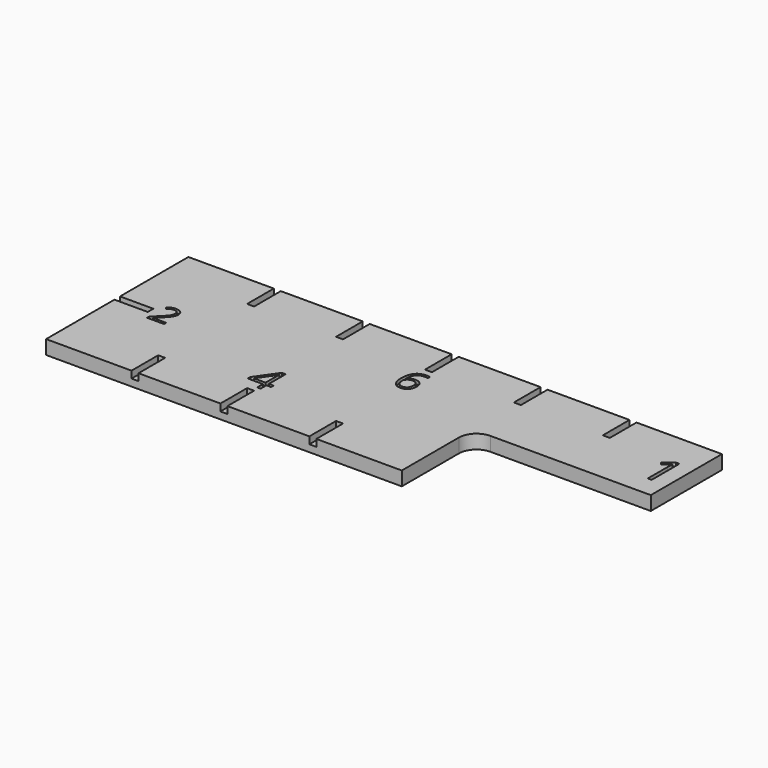
from build123d import *

# Parameters (mm, degrees)
F1_DEPTH       = 4
F3_DEPTH       = 2
F4_TEXT_SIZE   = 10.261640677
F4_TEXT_SIZE_2 = 11.3518313608
F4_TEXT_SIZE_3 = 12.4870120392
F4_TEXT_SIZE_4 = 13.8751825576
F5_DEPTH       = 1


# Not quite as in the source:
# - Text() gives the source's letters only with a copy of the font that has no kerning and outlines rounded to 1/6400 em; it was checked with that copy


with BuildPart() as f1:
    # F0 (on Top) → F1 (new body)
    with BuildSketch(Plane.XY):
        with BuildLine():
            Line((50.8, 25.4), (-50.8, 25.4))
            Line((-50.8, 25.4), (-50.8, -25.4))
            Line((-50.8, -25.4), (50.8, -25.4))
            Line((50.8, -25.4), (50.8, -5))
            ThreePointArc((50.8, -5), (52.2644660941, -1.4644660941), (55.8, 0))
            Line((55.8, 0), (101.6, 0))
            Line((101.6, 0), (101.6, 25.4))
            Line((101.6, 25.4), (50.8, 25.4))
        make_face()
    extrude(amount=F1_DEPTH)

    # F2 (on face) → F3 (cut)
    with BuildSketch(Plane.XY.offset(4)):
        Polygon((-1, 34.925), (-1, 25.4), (-1, 15.875), (1, 15.875), (1, 34.925), align=None)
        Polygon((-26.4, 15.875), (-24.4, 15.875), (-24.4, 25.4), (-24.4, 34.925), (-26.4, 34.925), (-26.4, 25.4), align=None)
        Polygon((24.4, 15.875), (26.4, 15.875), (26.4, 34.925), (24.4, 34.925), (24.4, 25.4), align=None)
        Polygon((75.2, 34.924999693), (75.2, 25.399999693), (75.2, 15.874999693), (77.2, 15.874999693), (77.2, 34.924999693), align=None)
        Polygon((49.8, 15.875), (51.8, 15.875), (51.8, 25.399999693), (51.8, 34.925), (49.8, 34.925), (49.8, 25.4), align=None)
        Polygon((-60.325, -0.999999693), (-50.8, -0.999999693), (-41.275, -0.999999693), (-41.275, 1.000000307), (-60.325, 1.000000307), align=None)
        Polygon((-0.9999993861, -15.875), (-0.9999993861, -25.4), (-0.9999993861, -34.925), (1.0000006139, -34.925), (1.0000006139, -15.875), align=None)
        Polygon((-26.3999993861, -15.875), (-26.3999993861, -25.4), (-26.3999993861, -34.925), (-24.3999993861, -34.925), (-24.3999993861, -25.4), (-24.3999993861, -15.875), align=None)
        Polygon((24.4000006139, -34.925), (26.4000006139, -34.925), (26.4000006139, -15.875), (24.4000006139, -15.875), (24.4000006139, -25.4), align=None)
    extrude(amount=-F3_DEPTH, mode=Mode.SUBTRACT)

    # F4 (on face) → F5 (cut)
    with BuildSketch(Plane.XY.offset(4)):
        with Locations((-40.1271991432, -3.2861479558)):
            Text('2', F4_TEXT_SIZE, font='Open Sans', text_align=(TextAlign.LEFT, TextAlign.BOTTOM))
        with Locations((22.1782419831, 5.68053592)):
            Text('6', F4_TEXT_SIZE_2, font='Open Sans', text_align=(TextAlign.LEFT, TextAlign.BOTTOM))
        with Locations((-4.0438554715, -14.207242988)):
            Text('4', F4_TEXT_SIZE_3, font='Open Sans', text_align=(TextAlign.LEFT, TextAlign.BOTTOM))
        with Locations((92.3000574112, 5.8848685585)):
            Text('1', F4_TEXT_SIZE_4, font='Open Sans', text_align=(TextAlign.LEFT, TextAlign.BOTTOM))
    extrude(amount=-F5_DEPTH, mode=Mode.SUBTRACT)


solid = f1.part
